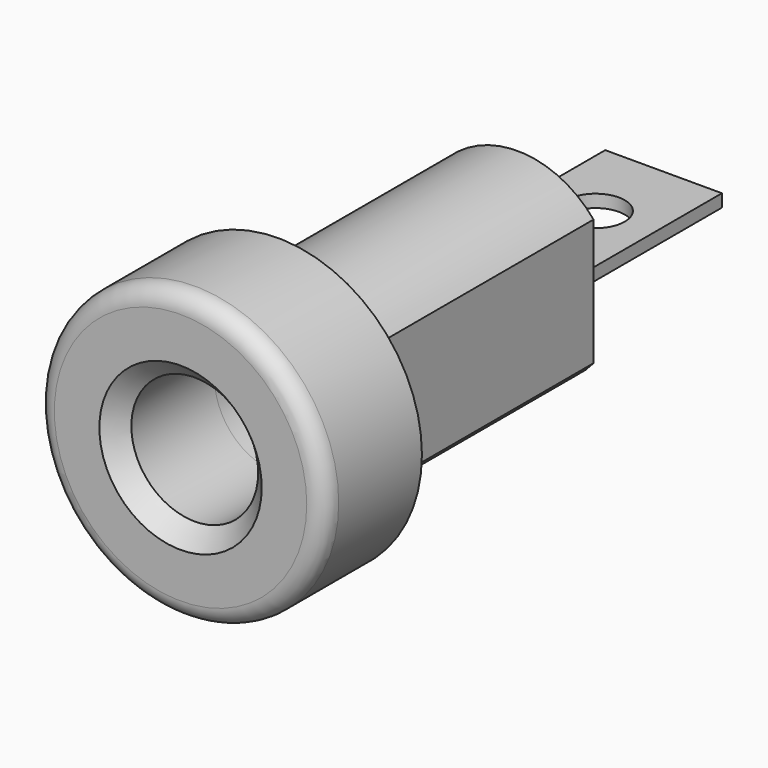
from build123d import *
from build123d import SkipClean  # not in build123d's __all__

# Parameters (mm, degrees)
F0_R      = 5.675
F0_R_2    = 2.5
F1_DEPTH  = 4.8
F2_R      = 0.7
F3_SIZE   = 0.7
F4_R      = 2.5
F5_DEPTH  = 11.7
F7_DEPTH  = 11
F9_DEPTH  = 0.1
F10_W     = 4.6
F10_H     = 0.5
F11_DEPTH = 7.2
F12_R     = 1.15
F13_DEPTH = 0.5


# Not quite as in the source:
# - after a boolean that leaves OpenCascade's solid faulty, fix() repairs it
# - a pattern or mirror of a feature is missing from the dataset's text; its kind, count and spacing are read off the source's solid


with BuildPart() as f1:
    # F0 (on Front) → F1 (new body)
    with BuildSketch(Plane.XZ):
        Circle(F0_R)
        Circle(F0_R_2, mode=Mode.SUBTRACT)
    extrude(amount=-F1_DEPTH)

    # F2
    f2_edges = [f1.edges().sort_by_distance(p)[0] for p in [
        (-5.675, 0, 0),
    ]]
    fillet(f2_edges, radius=F2_R)

    # F3
    f3_edges = [f1.edges().sort_by_distance(p)[0] for p in [
        (-2.5, 0, 0),
    ]]
    chamfer(f3_edges, length=F3_SIZE)

    # F4 (on face) → F5 (join)
    with BuildSketch(Plane(origin=(0, 4.8, 0), x_dir=(-1, 0, 0), z_dir=(0, 1, 0))):
        with BuildLine():
            Line((-3, 2.4919871589), (-3, -2.4919871589))
            ThreePointArc((-3, -2.4919871589), (0, -3.9), (3, -2.4919871589))
            Line((3, -2.4919871589), (3, 2.4919871589))
            ThreePointArc((3, 2.4919871589), (0, 3.9), (-3, 2.4919871589))
        make_face()
        Circle(F4_R, mode=Mode.SUBTRACT)
    with SkipClean():  # cleaning this boolean's faces spoils the solid; the shape is the same uncleaned
        extrude(amount=F5_DEPTH)

    # F6 (on face) → F7 (join)
    with BuildSketch(Plane(origin=(0, 16.5, 0), x_dir=(-1, 0, 0), z_dir=(0, 1, 0))):
        with BuildLine():
            Line((0.9797958971, 2.3), (-0.9797958971, 2.3))
            ThreePointArc((-0.9797958971, 2.3), (-1.767766953, 1.767766953), (-2.3, 0.9797958971))
            Line((-2.3, 0.9797958971), (-2.3, 0.68556546))
            Line((-2.3, 0.68556546), (-2.3, -0.9797958971))
            ThreePointArc((-2.3, -0.9797958971), (-1.767766953, -1.767766953), (-0.9797958971, -2.3))
            Line((-0.9797958971, -2.3), (0.9797958971, -2.3))
            ThreePointArc((0.9797958971, -2.3), (1.767766953, -1.767766953), (2.3, -0.9797958971))
            Line((2.3, -0.9797958971), (2.3, 0.9797958971))
            ThreePointArc((2.3, 0.9797958971), (1.767766953, 1.767766953), (0.9797958971, 2.3))
        make_face()
        with BuildLine():
            ThreePointArc((-2.2, 0.9591663047), (-1.6970562748, 1.6970562748), (-0.9591663047, 2.2))
            Line((-0.9591663047, 2.2), (0.9591663047, 2.2))
            ThreePointArc((0.9591663047, 2.2), (1.6970562748, 1.6970562748), (2.2, 0.9591663047))
            Line((2.2, 0.9591663047), (2.2, -0.9591663047))
            ThreePointArc((2.2, -0.9591663047), (1.6970562748, -1.6970562748), (0.9591663047, -2.2))
            Line((0.9591663047, -2.2), (-0.9591663047, -2.2))
            ThreePointArc((-0.9591663047, -2.2), (-1.6970562748, -1.6970562748), (-2.2, -0.9591663047))
            Line((-2.2, -0.9591663047), (-2.2, 0.9591663047))
        make_face(mode=Mode.SUBTRACT)
    extrude(amount=-F7_DEPTH)

    add(f1.part.fix(), mode=Mode.REPLACE)

    # F8 (on face) → F9 (join)
    with BuildSketch(Plane(origin=(0, 16.5, 0), x_dir=(-1, 0, 0), z_dir=(0, 1, 0))):
        with BuildLine():
            Line((3, -2.4919871589), (3, 2.4919871589))
            ThreePointArc((3, 2.4919871589), (0, 3.9), (-3, 2.4919871589))
            Line((-3, 2.4919871589), (-3, -2.4919871589))
            ThreePointArc((-3, -2.4919871589), (0, -3.9), (3, -2.4919871589))
        make_face()
        with BuildLine():
            ThreePointArc((0.9797958971, 2.3), (1.767766953, 1.767766953), (2.3, 0.9797958971))
            ThreePointArc((2.3, 0.9797958971), (2.4494897428, 0.5), (2.5, 0))
            ThreePointArc((2.5, 0), (2.4494897428, -0.5), (2.3, -0.9797958971))
            ThreePointArc((2.3, -0.9797958971), (1.767766953, -1.767766953), (0.9797958971, -2.3))
            ThreePointArc((0.9797958971, -2.3), (0, -2.5), (-0.9797958971, -2.3))
            ThreePointArc((-0.9797958971, -2.3), (-1.767766953, -1.767766953), (-2.3, -0.9797958971))
            ThreePointArc((-2.3, -0.9797958971), (-2.5, 0), (-2.3, 0.9797958971))
            ThreePointArc((-2.3, 0.9797958971), (-1.767766953, 1.767766953), (-0.9797958971, 2.3))
            ThreePointArc((-0.9797958971, 2.3), (0, 2.5), (0.9797958971, 2.3))
        make_face(mode=Mode.SUBTRACT)
        with BuildLine():
            Line((2.3, -0.9797958971), (2.3, 0.9797958971))
            ThreePointArc((2.3, 0.9797958971), (1.767766953, 1.767766953), (0.9797958971, 2.3))
            Line((0.9797958971, 2.3), (-0.9797958971, 2.3))
            ThreePointArc((-0.9797958971, 2.3), (-1.767766953, 1.767766953), (-2.3, 0.9797958971))
            Line((-2.3, 0.9797958971), (-2.3, -0.9797958971))
            ThreePointArc((-2.3, -0.9797958971), (-1.767766953, -1.767766953), (-0.9797958971, -2.3))
            Line((-0.9797958971, -2.3), (0.9797958971, -2.3))
            ThreePointArc((0.9797958971, -2.3), (1.767766953, -1.767766953), (2.3, -0.9797958971))
        make_face()
        with BuildLine():
            Line((-2.2, -0.9591663047), (-2.2, 0.9591663047))
            ThreePointArc((-2.2, 0.9591663047), (-1.6970562748, 1.6970562748), (-0.9591663047, 2.2))
            Line((-0.9591663047, 2.2), (0.9591663047, 2.2))
            ThreePointArc((0.9591663047, 2.2), (1.6970562748, 1.6970562748), (2.2, 0.9591663047))
            Line((2.2, 0.9591663047), (2.2, -0.9591663047))
            ThreePointArc((2.2, -0.9591663047), (1.6970562748, -1.6970562748), (0.9591663047, -2.2))
            Line((0.9591663047, -2.2), (-0.9591663047, -2.2))
            ThreePointArc((-0.9591663047, -2.2), (-1.6970562748, -1.6970562748), (-2.2, -0.9591663047))
        make_face(mode=Mode.SUBTRACT)
        with BuildLine():
            ThreePointArc((-0.9797958971, -2.3), (0, -2.5), (0.9797958971, -2.3))
            Line((0.9797958971, -2.3), (-0.9797958971, -2.3))
        make_face()
        with BuildLine():
            ThreePointArc((-0.9591663047, 2.2), (-1.6970562748, 1.6970562748), (-2.2, 0.9591663047))
            Line((-2.2, 0.9591663047), (-2.2, -0.9591663047))
            ThreePointArc((-2.2, -0.9591663047), (-1.6970562748, -1.6970562748), (-0.9591663047, -2.2))
            Line((-0.9591663047, -2.2), (0.9591663047, -2.2))
            ThreePointArc((0.9591663047, -2.2), (1.6970562748, -1.6970562748), (2.2, -0.9591663047))
            Line((2.2, -0.9591663047), (2.2, 0.9591663047))
            ThreePointArc((2.2, 0.9591663047), (1.6970562748, 1.6970562748), (0.9591663047, 2.2))
            Line((0.9591663047, 2.2), (-0.9591663047, 2.2))
        make_face()
        with BuildLine():
            ThreePointArc((2.5, 0), (2.4494897428, 0.5), (2.3, 0.9797958971))
            Line((2.3, 0.9797958971), (2.3, -0.9797958971))
            ThreePointArc((2.3, -0.9797958971), (2.4494897428, -0.5), (2.5, 0))
        make_face()
        with BuildLine():
            Line((-0.9797958971, 2.3), (0.9797958971, 2.3))
            ThreePointArc((0.9797958971, 2.3), (0, 2.5), (-0.9797958971, 2.3))
        make_face()
    f9 = extrude(amount=F9_DEPTH)

    # F9_copies: F9 across plane
    add(f9.mirror(Plane(origin=(0, 0, 0), x_dir=(0, 0, 1), z_dir=(1, 0, 0))), clean=False)

    # F10 (on face) → F11 (join)
    with BuildSketch(Plane(origin=(0, 16.6, 0), x_dir=(-1, 0, 0), z_dir=(0, 1, 0))):
        Rectangle(F10_W, F10_H)
    extrude(amount=F11_DEPTH)

    # F12 (on face) → F13 (cut)
    with BuildSketch(Plane(origin=(0, 0, -0.25), x_dir=(1, 0, 0), z_dir=(0, 0, -1))):
        with Locations((0, -20.45)):
            Circle(F12_R)
    extrude(amount=-F13_DEPTH, mode=Mode.SUBTRACT)


solid = f1.part
